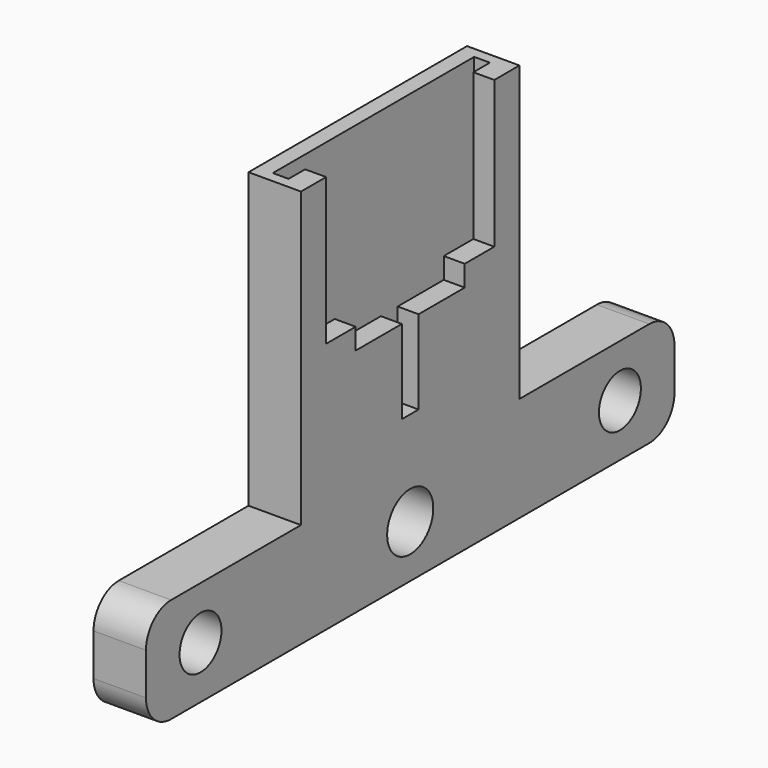
from build123d import *

# Parameters (mm, degrees)
F0_R     = 2.5
F1_DEPTH = 5
F2_D     = 5.5
F2_DEPTH = 7
F2_TIP   = 1.6523667023
F4_DEPTH = 5
F6_DEPTH = 3.5
F7_W     = 1.5
F7_H     = 1.975
F8_DEPTH = 24


with BuildPart() as f1:
    # F0 (on Right) → F1 (new body)
    with BuildSketch(Plane.YZ):
        with BuildLine():
            Line((-28.5, -5), (28.5, -5))
            ThreePointArc((28.5, -5), (30.6213203436, -4.1213203436), (31.5, -2))
            Line((31.5, -2), (31.5, 2))
            ThreePointArc((31.5, 2), (30.6213203436, 4.1213203436), (28.5, 5))
            Line((28.5, 5), (-28.5, 5))
            ThreePointArc((-28.5, 5), (-30.6213203436, 4.1213203436), (-31.5, 2))
            Line((-31.5, 2), (-31.5, -2))
            ThreePointArc((-31.5, -2), (-30.6213203436, -4.1213203436), (-28.5, -5))
        make_face()
        with Locations((-25, 0)):
            Circle(F0_R, mode=Mode.SUBTRACT)
        with Locations((25, 0)):
            Circle(F0_R, mode=Mode.SUBTRACT)
    extrude(amount=F1_DEPTH)

    # F2
    with Locations(Plane(origin=(0, 0, 0), x_dir=(0, 1, 0), z_dir=(-1, 0, 0))):
        with Locations((0, 0)):
            Hole(F2_D / 2, depth=F2_DEPTH)
            with Locations((0, 0, -(F2_DEPTH + F2_TIP / 2))):  # 118° drill point
                Cone(0, F2_D / 2, F2_TIP, mode=Mode.SUBTRACT)

    # F3 (on Right) → F4 (join, through all)
    with BuildSketch(Plane.YZ):
        Polygon((-13.025, 33), (-13.025, 5), (13.025, 5), (13.025, 33), (0, 33), align=None)
    extrude(amount=F4_DEPTH)

    # F5 (on face) → F6 (cut)
    with BuildSketch(Plane.YZ.offset(5)):
        Polygon((10.025, 33), (-10.025, 33), (-10.025, 19), (-6.5, 19), (-6.5, 17), (-1, 17), (-1, 9), (1, 9), (1, 17), (6.5, 17), (6.5, 19), (10.025, 19), align=None)
    extrude(amount=-F6_DEPTH, mode=Mode.SUBTRACT)

    # F7 (on face) → F8 (cut, through all)
    with BuildSketch(Plane.XY.offset(33)):
        Polygon((1.5, 10.025), (1.5, 0), (1.5, -10.025), (3, -10.025), (3, 0), (3, 10.025), align=None)
        with Locations((2.25, -11.0125)):
            Rectangle(F7_W, F7_H)
        with Locations((2.25, 11.0125)):
            Rectangle(F7_W, F7_H)
    extrude(amount=-F8_DEPTH, mode=Mode.SUBTRACT)


solid = f1.part
